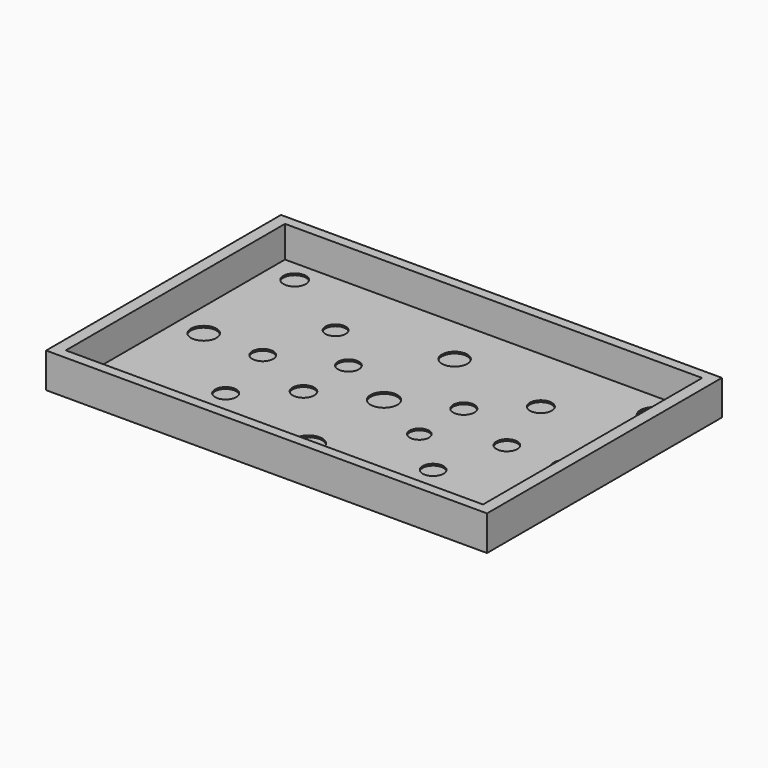
from build123d import *

# Parameters (mm, degrees)
F0_W      = 126.2549012899
F0_H      = 84.0705931187
F1_DEPTH  = 10
F2_W      = 119.4519400597
F2_H      = 78.4470066428
F3_DEPTH  = 9
F6_R      = 2.7574274492
F6_R_2    = 3.0881184617
F6_R_3    = 2.9865161703
F7_DEPTH  = 9.5
F5_R      = 3.0287162896
F8_DEPTH  = 9.5
F4_R      = 3.8384708655
F9_DEPTH  = 9.5
F10_R     = 3.132111717
F10_R_2   = 2.9916448853
F10_R_3   = 3.0367007185
F10_R_4   = 2.8900379759
F11_DEPTH = 9.5
F13_R     = 3.0036385534
F13_R_2   = 2.9794176667
F13_R_3   = 3.6399459422
F13_R_4   = 3.1255773117
F14_DEPTH = 9.5
F12_R     = 3.2154485225
F12_R_2   = 2.6789056155
F12_R_3   = 3.0133824395
F12_R_4   = 3.8856724273
F15_DEPTH = 9.5
F16_R     = 3.6323450942
F16_R_2   = 3.9223279678
F17_DEPTH = 9.5


# Not quite as in the source:
# - a feature names something its author has since deleted; it is built from what else it names


with BuildPart() as f1:
    # F0 (on Top) → F1 (new body)
    with BuildSketch(Plane.XY):
        Rectangle(F0_W, F0_H)
    extrude(amount=-F1_DEPTH)

    # F2 (on Top) → F3 (cut)
    with BuildSketch(Plane.XY):
        Rectangle(F2_W, F2_H)
    extrude(amount=-F3_DEPTH, mode=Mode.SUBTRACT)

    # F6 (on Top) → F7 (cut)
    with BuildSketch(Plane.XY):
        with Locations((16.5214389563, -8.0118775368)):
            Circle(F6_R)
        with Locations((-16.615998, -8.0534629524)):
            Circle(F6_R_2)
        with Locations((-16.615998, 8.0431699753)):
            Circle(F6_R_3)
    extrude(amount=-F7_DEPTH, mode=Mode.SUBTRACT)

    # F5 (on Top) → F8 (cut)
    with BuildSketch(Plane.XY):
        with Locations((16.5819376707, 7.8347064555)):
            Circle(F5_R)
    extrude(amount=-F8_DEPTH, mode=Mode.SUBTRACT)

    # F4 (on Top) → F9 (cut)
    with BuildSketch(Plane.XY):
        Circle(F4_R)
    extrude(amount=-F9_DEPTH, mode=Mode.SUBTRACT)

    # F10 (on face) → F11 (cut)
    with BuildSketch(Plane.XY):
        with Locations((29.441639781, 19.3310081959)):
            Circle(F10_R)
        with Locations((29.7522768378, -19.6110159159)):
            Circle(F10_R_2)
        with Locations((-29.6404287219, -19.6110159159)):
            Circle(F10_R_3)
        with Locations((-29.5161753893, 19.5709131658)):
            Circle(F10_R_4)
    extrude(amount=-F11_DEPTH, mode=Mode.SUBTRACT)

    # F13 (on Top) → F14 (cut)
    with BuildSketch(Plane.XY):
        with Locations((-34.714885056, 0)):
            Circle(F13_R)
        with Locations((35.1781696081, 0)):
            Circle(F13_R_2)
        with Locations((-51.6325049102, 0)):
            Circle(F13_R_3)
        with Locations((51.6923218966, 0)):
            Circle(F13_R_4)
    extrude(amount=-F14_DEPTH, mode=Mode.SUBTRACT)

    # F12 (on Top) → F15 (cut)
    with BuildSketch(Plane.XY):
        with Locations((-51.8871918321, 32.8838564456)):
            Circle(F12_R)
        with Locations((-51.9447661936, -32.4058681726)):
            Circle(F12_R_2)
        with Locations((51.5429228544, -32.7062048018)):
            Circle(F12_R_3)
        with Locations((51.7358258367, 31.9894589484)):
            Circle(F12_R_4)
    extrude(amount=-F15_DEPTH, mode=Mode.SUBTRACT)

    # F16 (on Top) → F17 (cut)
    with BuildSketch(Plane.XY):
        with Locations((0, 25.2807121724)):
            Circle(F16_R)
        with Locations((0, -27.0220451057)):
            Circle(F16_R_2)
    extrude(amount=-F17_DEPTH, mode=Mode.SUBTRACT)


solid = f1.part
